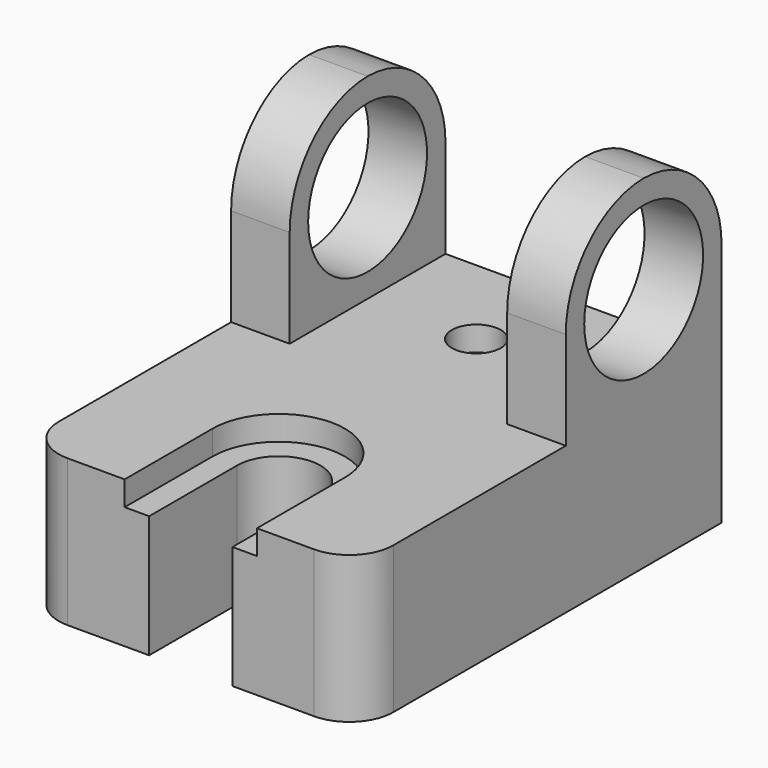
from build123d import *

# Parameters (mm, degrees)
F1_DEPTH        = 25
F2_DEPTH        = 30
F3_W            = 11.9576826692
F3_H            = 39.7608936764
F4_DEPTH        = 40
F5_R            = 15.1725757167
F6_DEPTH        = 68.3238299022
F7_T1_DEPTH     = 111.9576826692
F7_T3_DEPTH     = 111.9576826692
F8_R            = 9
F10_D           = 8
F10_DEPTH       = 10
F10_CBORE_D     = 10
F10_CBORE_DEPTH = 5
F10_TIP         = 2.4034424761


# Not quite as in the source:
# - a fillet or chamfer that OpenCascade refuses, or shapes differently, is made with other operations: its cross-section is extruded or revolved along the edge and cut away or added


with BuildPart() as f1:
    # F0 (on Top) → F1 (new body)
    with BuildSketch(Plane.XY):
        with BuildLine():
            Line((8.5056748986, -46.3761053979), (13.5056748986, -46.3761053979))
            Line((13.5056748986, -46.3761053979), (13.5056748986, -23.932851851))
            ThreePointArc((13.5056748986, -23.932851851), (0, -10.4271769524), (-13.5056748986, -23.932851851))
            Line((-13.5056748986, -23.932851851), (-13.5056748986, -46.3761053979))
            Line((-13.5056748986, -46.3761053979), (-8.5056748986, -46.3761053979))
            Line((-8.5056748986, -46.3761053979), (-8.5056748986, -23.932851851))
            ThreePointArc((-8.5056748986, -23.932851851), (0, -15.4271769524), (8.5056748986, -23.932851851))
            Line((8.5056748986, -23.932851851), (8.5056748986, -46.3761053979))
        make_face()
    extrude(amount=F1_DEPTH)

    # F0 (on Top) → F2 (join)
    with BuildSketch(Plane.XY):
        with BuildLine():
            Line((34.1614149511, -46.3761053979), (34.1614149511, 46.3761053979))
            Line((34.1614149511, 46.3761053979), (-34.1614149511, 46.3761053979))
            Line((-34.1614149511, 46.3761053979), (-34.1614149511, -46.3761053979))
            Line((-34.1614149511, -46.3761053979), (-13.5056748986, -46.3761053979))
            Line((-13.5056748986, -46.3761053979), (-13.5056748986, -23.932851851))
            ThreePointArc((-13.5056748986, -23.932851851), (0, -10.4271769524), (13.5056748986, -23.932851851))
            Line((13.5056748986, -23.932851851), (13.5056748986, -46.3761053979))
            Line((13.5056748986, -46.3761053979), (34.1614149511, -46.3761053979))
        make_face()
    extrude(amount=F2_DEPTH)

    # F3 (on face) → F4 (join)
    with BuildSketch(Plane.XY.offset(30)):
        with Locations((28.1825736165, 26.4956585597)):
            Rectangle(F3_W, F3_H)
        with Locations((-28.1825736165, 26.4956585597)):
            Rectangle(F3_W, F3_H)
    extrude(amount=F4_DEPTH)

    # F5 (on face) → F6 (cut, through all)
    with BuildSketch(Plane(origin=(-34.1614149511, 0, 0), x_dir=(0, -1, 0), z_dir=(-1, 0, 0))):
        with Locations((-26.4956585597, 50)):
            Circle(F5_R)
    extrude(amount=-F6_DEPTH, mode=Mode.SUBTRACT)

    # F7: fillet of radius 20 on 4 edges, made by hand

    # F7_s2 → F7_t1 (cut)
    with BuildSketch(Plane.YZ.offset(-84.1614149511)):
        with BuildLine():
            ThreePointArc((6.6152117215, 50), (12.4730760978, 64.1421356237), (26.6152117215, 70))
            Line((26.6152117215, 70), (6.6152117215, 70))
            Line((6.6152117215, 70), (6.6152117215, 50))
        make_face()
        with BuildLine():
            ThreePointArc((46.3761053979, 50), (40.5182410217, 64.1421356237), (26.3761053979, 70))
            Line((26.3761053979, 70), (46.3761053979, 70))
            Line((46.3761053979, 70), (46.3761053979, 50))
        make_face()
    extrude(amount=F7_T1_DEPTH, mode=Mode.SUBTRACT)

    # F7_s4 → F7_t3 (cut)
    with BuildSketch(Plane.YZ.offset(-27.7962677181)):
        with BuildLine():
            ThreePointArc((6.6152117215, 50), (12.4730760978, 64.1421356237), (26.6152117215, 70))
            Line((26.6152117215, 70), (6.6152117215, 70))
            Line((6.6152117215, 70), (6.6152117215, 50))
        make_face()
        with BuildLine():
            ThreePointArc((46.3761053979, 50), (40.5182410217, 64.1421356237), (26.3761053979, 70))
            Line((26.3761053979, 70), (46.3761053979, 70))
            Line((46.3761053979, 70), (46.3761053979, 50))
        make_face()
    extrude(amount=F7_T3_DEPTH, mode=Mode.SUBTRACT)

    # F8
    f8_edges = [f1.edges().sort_by_distance(p)[0] for p in [
        (34.161415, -46.376105, 15),
        (-34.161415, -46.376105, 15),
    ]]
    fillet(f8_edges, radius=F8_R)

    # F10
    with Locations(Plane.XY.offset(30)):
        with Locations((0, 26.4956585597)):
            CounterBoreHole(F10_D / 2, F10_CBORE_D / 2, F10_CBORE_DEPTH, depth=F10_DEPTH)
            with Locations((0, 0, -(F10_DEPTH + F10_TIP / 2))):  # 118° drill point
                Cone(0, F10_D / 2, F10_TIP, mode=Mode.SUBTRACT)


solid = f1.part
